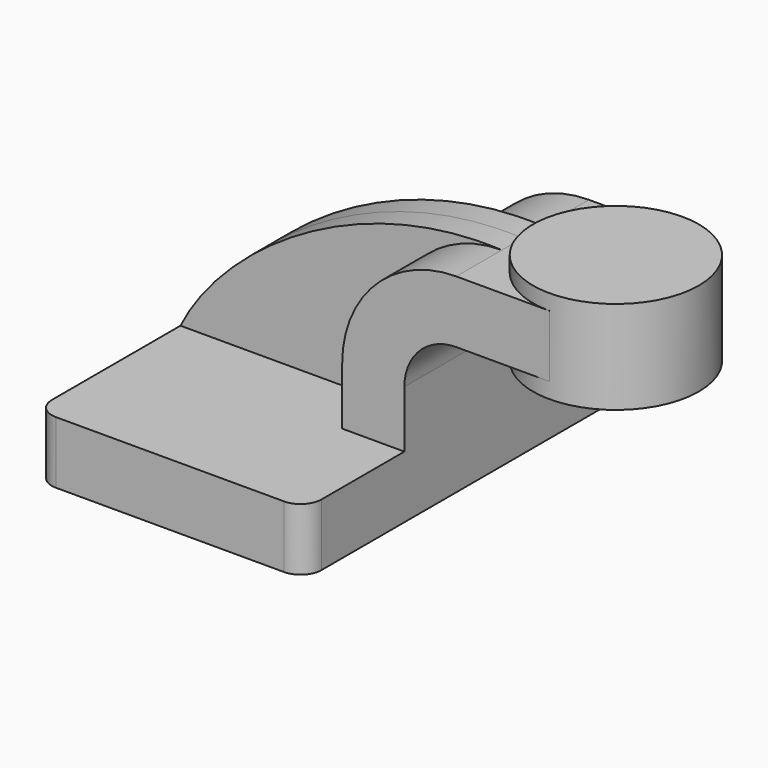
from build123d import *

# Parameters (mm, degrees)
F1_DEPTH = 63.5
F0_W     = 25.4
F0_H     = 19.05
F2_DEPTH = 25.4
F3_DEPTH = 7.9375
F5_R     = 6.35


# Not quite as in the source:
# - ends of sketch curves that miss each other by under 0.0002 mm in the source are joined


with BuildPart() as f1:
    # F0 (on Front) → F1 (new body, symmetric)
    with BuildSketch(Plane.XZ):
        Polygon((-41.275, -9.525), (41.275, -9.525), (41.275, 9.525), (22.225, 9.525), (-41.275, 9.525), align=None)
    extrude(amount=F1_DEPTH, both=True)

    # F0 (on Front) → F2 (join, symmetric)
    with BuildSketch(Plane.XZ):
        with BuildLine():
            Line((22.225, 9.525), (41.275, 9.525))
            Line((41.275, 9.525), (41.275, 27.0002))
            ThreePointArc((41.275, 27.0002), (45.9246798487, 38.2255201513), (57.15, 42.8752))
            Line((57.15, 42.8752), (60.325, 42.8752))
            Line((60.325, 42.8752), (60.325, 61.9252))
            Line((60.325, 61.9252), (57.15, 61.9252))
            ThreePointArc((57.15, 61.9252), (32.4542956671, 51.6959043329), (22.225, 27.0002))
            Line((22.225, 27.0002), (22.225, 9.525))
        make_face()
        with Locations((73.025, 52.4002)):
            Rectangle(F0_W, F0_H)
    extrude(amount=F2_DEPTH, both=True)

    # F0 (on Front) → F3 (join, symmetric)
    with BuildSketch(Plane.XZ):
        with BuildLine():
            add(Edge.make_bspline(
                [(-41.275, 9.525), (-28.5102911294, 35.4532189667), (11.965462938, 64.1112402081), (57.15, 61.9252)],
                knots=[0, 0, 0, 0, 111.5045361635, 111.5045361635, 111.5045361635, 111.5045361635], degree=3))
            Line((-41.275, 9.525), (22.225, 9.525))
            Line((22.225, 9.525), (22.225, 27.0002))
            ThreePointArc((22.225, 27.0002), (32.4542956671, 51.6959043329), (57.15, 61.9252))
        make_face()
    extrude(amount=F3_DEPTH, both=True)

    # F5
    f5_edges = [f1.edges().sort_by_distance(p)[0] for p in [
        (41.275, -63.5, 0),
        (-41.275, -63.5, 0),
        (41.275, 63.5, 0),
        (-41.275, 63.5, 0),
    ]]
    fillet(f5_edges, radius=F5_R)


with BuildPart() as f4:
    # F0 (on Front) → F4 (revolve)
    with BuildSketch(Plane.XZ):
        Polygon((85.725, 66.675), (85.725, 61.9252), (85.725, 42.8752), (85.725, 38.1), (111.125, 38.1), (111.125, 66.675), align=None)
    revolve(axis=Axis((85.725, 0, 52.3875), (0, 0, 1)))


solid = Compound([f1.part, f4.part])
